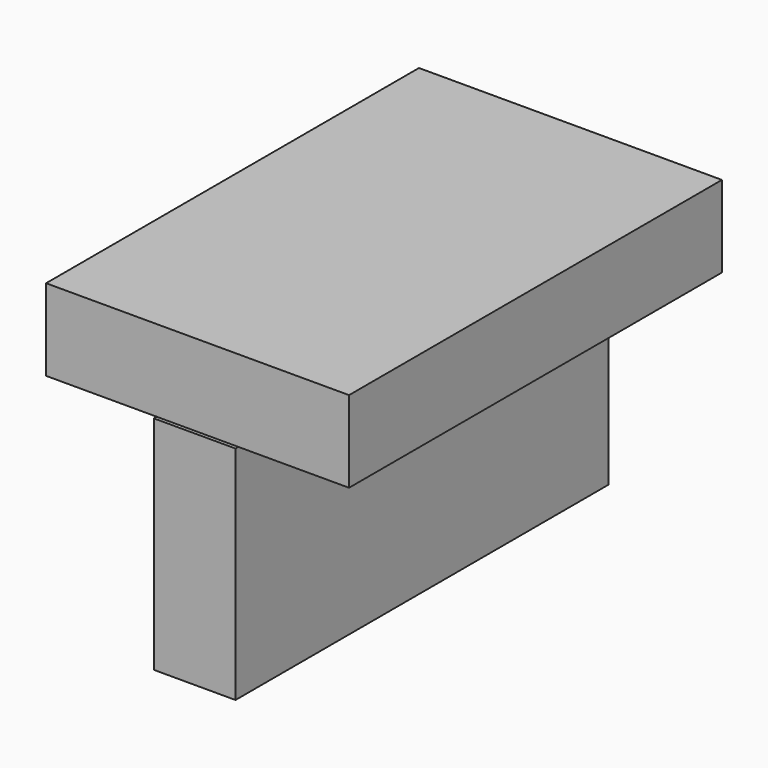
from build123d import *

# Parameters (mm, degrees)
F1_W     = 26
F1_H     = 40
F2_DEPTH = 7
F0_W     = 40
F0_H     = 19
F3_DEPTH = 3.5


with BuildPart() as f2:
    # F1 (on Top) → F2 (new body)
    with BuildSketch(Plane.XY):
        Rectangle(F1_W, F1_H)
    extrude(amount=F2_DEPTH)

    # F0 (on Right) → F3 (join, symmetric)
    with BuildSketch(Plane.YZ):
        with Locations((-0.3058470263, -9.5)):
            Rectangle(F0_W, F0_H)
    extrude(amount=F3_DEPTH, both=True)


solid = f2.part
